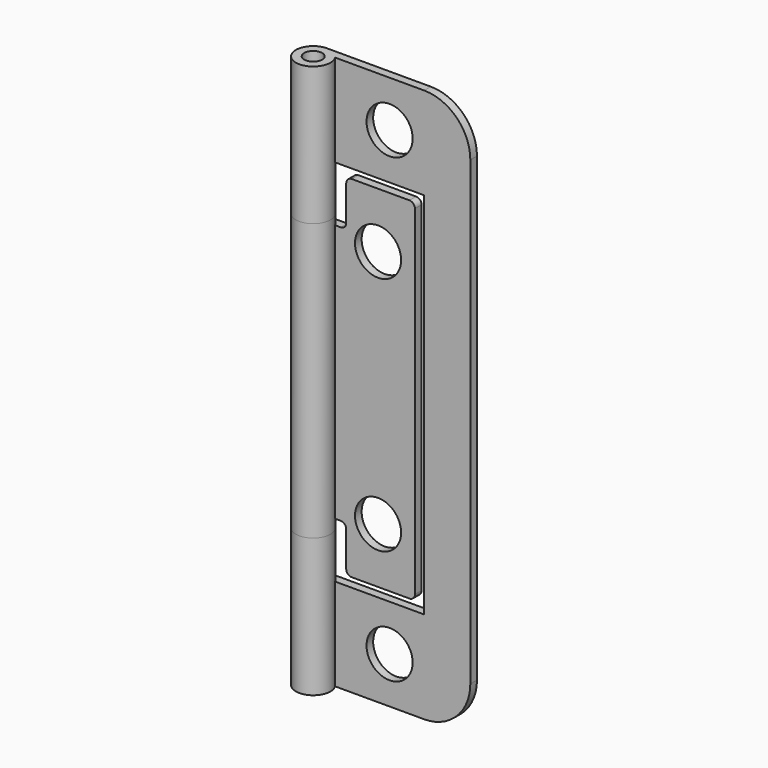
from build123d import *

# Parameters (mm, degrees)
F1_R     = 3.175
F2_DEPTH = 0.5715
F3_R     = 2.38125
F3_R_2   = 1.23825
F4_DEPTH = 19.05
F6_R     = 2.38125
F6_R_2   = 1.23825
F7_DEPTH = 38.1
F8_R     = 3.175
F9_DEPTH = 0.5715


# Not quite as in the source:
# - a pattern or mirror of a feature is missing from the dataset's text; its kind, count and spacing are read off the source's solid


with BuildPart() as f2:
    # F1 (on Front) → F2 (new body, symmetric)
    with BuildSketch(Plane.XZ):
        with BuildLine():
            Line((0, 12.7), (0, 0))
            Line((0, 0), (14.2875, 0))
            ThreePointArc((14.2875, 0), (18.7776280605, 1.8598719395), (20.6375, 6.35))
            Line((20.6375, 6.35), (20.6375, 69.85))
            ThreePointArc((20.6375, 69.85), (18.7776280605, 74.3401280605), (14.2875, 76.2))
            Line((14.2875, 76.2), (0, 76.2))
            Line((0, 76.2), (0, 63.5))
            Line((0, 63.5), (14.2875, 63.5))
            Line((14.2875, 63.5), (14.2875, 12.7))
            Line((14.2875, 12.7), (0, 12.7))
        make_face()
        with Locations((9.525, 6.35)):
            Circle(F1_R, mode=Mode.SUBTRACT)
        with Locations((9.525, 69.85)):
            Circle(F1_R, mode=Mode.SUBTRACT)
    extrude(amount=F2_DEPTH, both=True)

    # F3 (on face) → F4 (join)
    with BuildSketch(Plane.XY.offset(76.2)):
        with Locations((0, -1.80975)):
            Circle(F3_R)
        with Locations((0, -1.80975)):
            Circle(F3_R_2, mode=Mode.SUBTRACT)
    f4 = extrude(amount=-F4_DEPTH)

    # F4_copies: F4 across plane
    add(f4.mirror(Plane(origin=(0, 0, 38.1), x_dir=(-1, 0, 0), z_dir=(0, 0, -1))))


with BuildPart() as f7:
    # F6 (on face) → F7 (new body)
    with BuildSketch(Plane(origin=(0, 0, 57.15), x_dir=(1, 0, 0), z_dir=(0, 0, -1))):
        with Locations((0, 1.80975)):
            Circle(F6_R)
        with Locations((0, 1.80975)):
            Circle(F6_R_2, mode=Mode.SUBTRACT)
    extrude(amount=F7_DEPTH)

    # F8 (on Front) → F9 (join, symmetric)
    with BuildSketch(Plane.XZ):
        with BuildLine():
            Line((12.2555, 62.23), (4.318, 62.23))
            ThreePointArc((4.318, 62.23), (3.7791846327, 62.0068153673), (3.556, 61.468))
            Line((3.556, 61.468), (3.556, 56.642))
            ThreePointArc((3.556, 56.642), (3.3328153673, 56.1031846327), (2.794, 55.88))
            Line((2.794, 55.88), (0, 55.88))
            Line((0, 55.88), (0, 20.32))
            Line((0, 20.32), (2.794, 20.32))
            ThreePointArc((2.794, 20.32), (3.3328153673, 20.0968153673), (3.556, 19.558))
            Line((3.556, 19.558), (3.556, 14.732))
            ThreePointArc((3.556, 14.732), (3.7791846327, 14.1931846327), (4.318, 13.97))
            Line((4.318, 13.97), (12.2555, 13.97))
            ThreePointArc((12.2555, 13.97), (12.7943153673, 14.1931846327), (13.0175, 14.732))
            Line((13.0175, 14.732), (13.0175, 61.468))
            ThreePointArc((13.0175, 61.468), (12.7943153673, 62.0068153673), (12.2555, 62.23))
        make_face()
        with Locations((7.9375, 21.59)):
            Circle(F8_R, mode=Mode.SUBTRACT)
        with Locations((7.9375, 54.61)):
            Circle(F8_R, mode=Mode.SUBTRACT)
    extrude(amount=F9_DEPTH, both=True)


solid = Compound([f2.part, f7.part])
